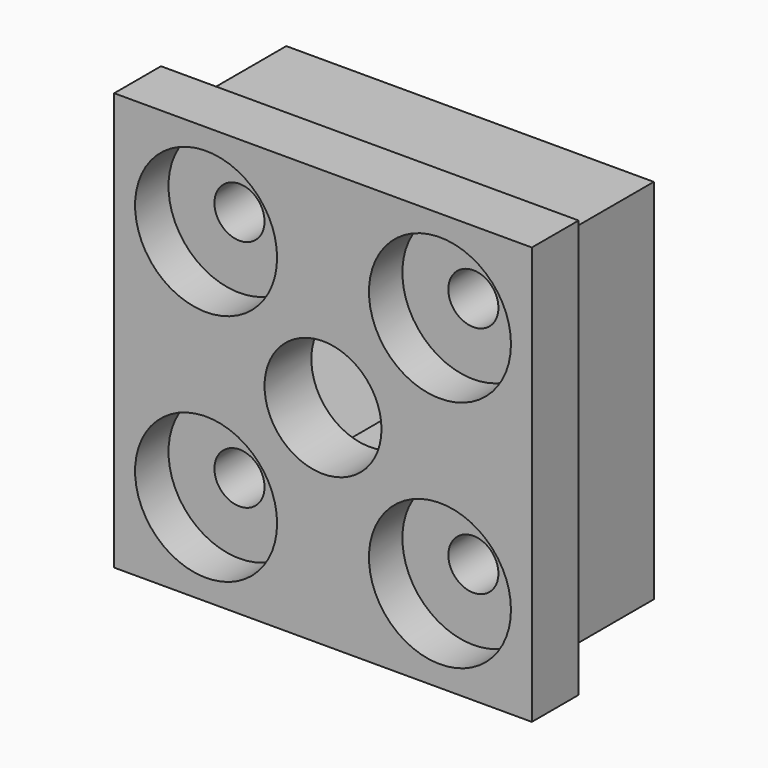
from build123d import *

# Parameters (mm, degrees)
F0_W      = 50
F0_H      = 50
F1_DEPTH  = 7
F2_W      = 44
F2_H      = 44
F3_DEPTH  = 15
F4_R      = 3
F5_DEPTH  = 25
F7_R      = 7
F8_DEPTH  = 25
F9_R      = 7
F10_DEPTH = 15
F6_R      = 8.5
F11_DEPTH = 5


# Not quite as in the source:
# - a feature names something its author has since deleted; it is built from what else it names


with BuildPart() as f1:
    # F0 (on Front) → F1 (new body)
    with BuildSketch(Plane.XZ):
        Rectangle(F0_W, F0_H)
    extrude(amount=-F1_DEPTH)

    # F2 (on face) → F3 (join)
    with BuildSketch(Plane(origin=(0, 7, 0), x_dir=(-1, 0, 0), z_dir=(0, 1, 0))):
        Rectangle(F2_W, F2_H)
    extrude(amount=F3_DEPTH)

    # F4 (on face) → F5 (cut)
    with BuildSketch(Plane(origin=(0, 22, 0), x_dir=(-1, 0, 0), z_dir=(0, 1, 0))):
        with Locations((-14, 14)):
            Circle(F4_R)
        with Locations((14, 14)):
            Circle(F4_R)
        with Locations((14, -14)):
            Circle(F4_R)
        with Locations((-14, -14)):
            Circle(F4_R)
    extrude(amount=-F5_DEPTH, mode=Mode.SUBTRACT)

    # F7 (on face) → F8 (cut)
    with BuildSketch(Plane.XZ):
        Circle(F7_R)
    extrude(amount=-F8_DEPTH, mode=Mode.SUBTRACT)

    # F9 (on face) → F10 (cut)
    with BuildSketch(Plane(origin=(0, 22, 0), x_dir=(-1, 0, 0), z_dir=(0, 1, 0))):
        Polygon((-5.4848275573, -9.5), (5.4848275573, -9.5), (10.9696551146, 0), (5.4848275573, 9.5), (-5.4848275573, 9.5), (-10.9696551146, 0), align=None)
        Circle(F9_R, mode=Mode.SUBTRACT)
    extrude(amount=-F10_DEPTH, mode=Mode.SUBTRACT)

    # F6 (on face) → F11 (cut)
    with BuildSketch(Plane.XZ):
        with Locations((-14, 14)):
            Circle(F6_R)
        with Locations((-14, -14)):
            Circle(F6_R)
        with Locations((14, -14)):
            Circle(F6_R)
        with Locations((14, 14)):
            Circle(F6_R)
    extrude(amount=-F11_DEPTH, mode=Mode.SUBTRACT)


solid = f1.part
